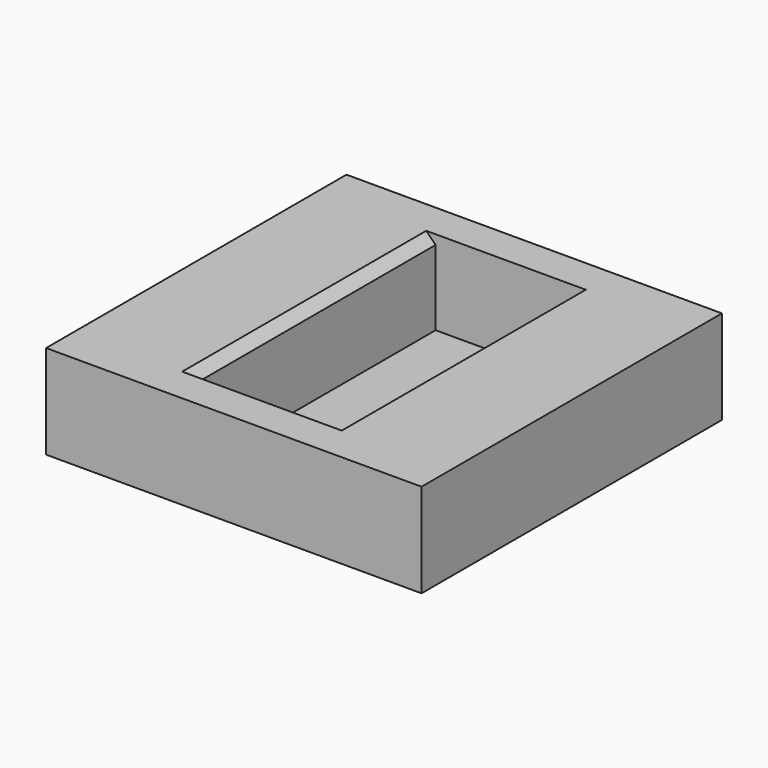
from build123d import *

# Parameters (mm, degrees)
F0_W     = 203.2
F0_H     = 203.2
F0_W_2   = 76.2
F0_H_2   = 165.1
F1_DEPTH = 5.08
F2_DEPTH = 50.8
F3_SIZE  = 5.08


with BuildPart() as f1:
    # F0 (on Top) → F1 (new body)
    with BuildSketch(Plane.XY):
        Rectangle(F0_W, F0_H)
        Rectangle(F0_W_2, F0_H_2, mode=Mode.SUBTRACT)
        Rectangle(F0_W_2, F0_H_2)
    extrude(amount=F1_DEPTH)

    # F0 (on Top) → F2 (join)
    with BuildSketch(Plane.XY):
        Rectangle(F0_W, F0_H)
        Rectangle(F0_W_2, F0_H_2, mode=Mode.SUBTRACT)
    extrude(amount=F2_DEPTH)

    # F3
    f3_edges = [f1.edges().sort_by_distance(p)[0] for p in [
        (-38.1, 0, 50.8),
        (38.1, 0, 50.8),
    ]]
    chamfer(f3_edges, length=F3_SIZE)


solid = f1.part
